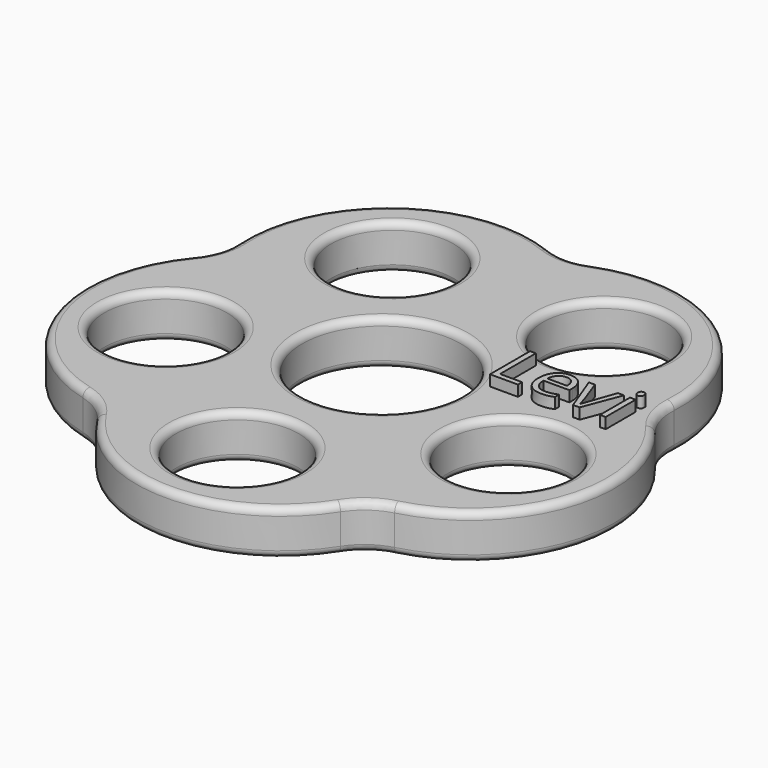
from build123d import *

# Parameters (mm, degrees)
F0_R         = 8.5
F0_R_2       = 11
F1_DEPTH     = 6.2
F2_R         = 8
F3_R         = 1
F4_TEXT_SIZE = 9.7222222222
F5_DEPTH     = 1.5
F6_TEXT_SIZE = 6.9444444444
F7_DEPTH     = 0.5


# Not quite as in the source:
# - Text() gives the source's letters only with a copy of the font that has no kerning and outlines rounded to 1/6400 em; it was checked with that copy


with BuildPart() as f1:
    # F0 (on Top) → F1 (new body)
    with BuildSketch(Plane.XY):
        with BuildLine():
            ThreePointArc((29.7774457087, 9.6752786143), (22.041946961, 30.3381372891), (0, 31.309859297))
            ThreePointArc((0, 31.309859297), (-22.041946961, 30.3381372891), (-29.7774457087, 9.6752786142))
            ThreePointArc((-29.7774457087, 9.6752786142), (-35.6646193611, -11.5881372891), (-18.4034735461, -25.3302082627))
            ThreePointArc((-18.4034735461, -25.3302082627), (0, -37.5), (18.4034735461, -25.3302082627))
            ThreePointArc((18.4034735461, -25.3302082627), (35.6646193611, -11.5881372891), (29.7774457087, 9.6752786143))
        make_face()
        with Locations((0, -25)):
            Circle(F0_R, mode=Mode.SUBTRACT)
        with Locations((-23.7764129074, -7.7254248594)):
            Circle(F0_R, mode=Mode.SUBTRACT)
        with Locations((23.7764129074, -7.7254248594)):
            Circle(F0_R, mode=Mode.SUBTRACT)
        Circle(F0_R_2, mode=Mode.SUBTRACT)
        with Locations((-14.6946313073, 20.2254248594)):
            Circle(F0_R, mode=Mode.SUBTRACT)
        with Locations((14.6946313073, 20.2254248594)):
            Circle(F0_R, mode=Mode.SUBTRACT)
    extrude(amount=F1_DEPTH)

    # F2
    f2_edges = [f1.edges().sort_by_distance(p)[0] for p in [
        (18.403474, -25.330208, 3.1),
        (29.777446, 9.675279, 3.1),
        (0, 31.309859, 3.1),
        (-29.777446, 9.675279, 3.1),
        (-18.403474, -25.330208, 3.1),
    ]]
    fillet(f2_edges, radius=F2_R)

    # F3
    f3_edges = [f1.edges().sort_by_distance(p)[0] for p in [
        (0, -37.5, 6.2),
        (-18.92665, -26.050299, 6.2),
        (18.92665, -26.050299, 6.2),
        (-35.664619, -11.588137, 6.2),
        (35.664619, -11.588137, 6.2),
        (-30.623963, 9.950329, 6.2),
        (30.623963, 9.950329, 6.2),
        (-22.041947, 30.338137, 6.2),
        (22.041947, 30.338137, 6.2),
        (0, 32.199941, 6.2),
        (-8.5, -25, 6.2),
        (-32.276413, -7.725425, 6.2),
        (15.276413, -7.725425, 6.2),
        (-11, 0, 6.2),
        (-23.194631, 20.225425, 6.2),
        (6.194631, 20.225425, 6.2),
        (0, -37.5, 0),
        (-18.92665, -26.050299, 0),
        (18.92665, -26.050299, 0),
        (-35.664619, -11.588137, 0),
        (35.664619, -11.588137, 0),
        (-30.623963, 9.950329, 0),
        (30.623963, 9.950329, 0),
        (-22.041947, 30.338137, 0),
        (22.041947, 30.338137, 0),
        (0, 32.199941, 0),
        (-8.5, -25, 0),
        (-32.276413, -7.725425, 0),
        (15.276413, -7.725425, 0),
        (-11, 0, 0),
        (-23.194631, 20.225425, 0),
        (6.194631, 20.225425, 0),
    ]]
    fillet(f3_edges, radius=F3_R)

    # F4 (on face) → F5 (join)
    with BuildSketch(Plane.XY.offset(6.2)):
        with Locations((11.4100779076, 3.3472230836)):
            Text('Levi', F4_TEXT_SIZE, font='Open Sans', text_align=(TextAlign.LEFT, TextAlign.BOTTOM))
    extrude(amount=F5_DEPTH)

    # F6 (on face) → F7 (cut)
    with BuildSketch(Plane(origin=(0, 0, 0), x_dir=(1, 0, 0), z_dir=(0, 0, -1))):
        with Locations((-30.0311414931, -6.2623811968)):
            Text('Jesus              Loves', F6_TEXT_SIZE, font='Open Sans', text_align=(TextAlign.LEFT, TextAlign.BOTTOM))
        with Locations((-7.0643446181, -29.7959150001)):
            Text('You!', F6_TEXT_SIZE, font='Open Sans', text_align=(TextAlign.LEFT, TextAlign.BOTTOM))
    extrude(amount=-F7_DEPTH, mode=Mode.SUBTRACT)


solid = f1.part
